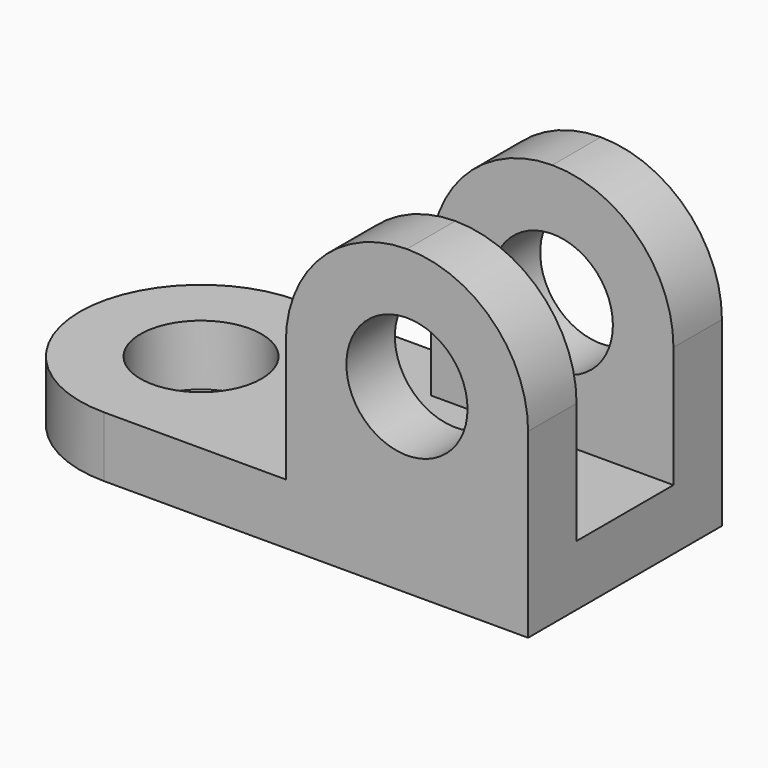
from build123d import *

# Parameters (mm, degrees)
F0_W      = 114.3
F0_H      = 63.5
F1_DEPTH  = 50.8
F2_W      = 25.4
F2_H      = 57.0441053795
F3_DEPTH  = 114.301
F4_W      = 63.5
F4_H      = 12.7
F5_DEPTH  = 50.8
F6_W      = 63.5
F6_H      = 12.7
F7_DEPTH  = 50.8
F8_R      = 12.7
F9_DEPTH  = 50.801
F10_R     = 25.39999
F11_R     = 12.7
F12_DEPTH = 12.701


# Not quite as in the source:
# - a fillet or chamfer is up to 0.001 mm smaller than in the source, because OpenCascade refuses the exact size


with BuildPart() as f1:
    # F0 (on Front) → F1 (new body)
    with BuildSketch(Plane.XZ):
        with Locations((5.5195242167, 20.4444855223)):
            Rectangle(F0_W, F0_H)
    extrude(amount=F1_DEPTH)

    # F2 (on face) → F3 (cut, through all)
    with BuildSketch(Plane.YZ.offset(62.6695242167)):
        with Locations((-25.4, 29.9165382121)):
            Rectangle(F2_W, F2_H)
    extrude(amount=-F3_DEPTH, mode=Mode.SUBTRACT)

    # F4 (on face) → F5 (cut)
    with BuildSketch(Plane.XY.offset(52.1944855223)):
        with Locations((-19.8804757833, -44.45)):
            Rectangle(F4_W, F4_H)
    extrude(amount=-F5_DEPTH, mode=Mode.SUBTRACT)

    # F6 (on face) → F7 (cut)
    with BuildSketch(Plane.XY.offset(52.1944855223)):
        with Locations((-19.8804757833, -6.35)):
            Rectangle(F6_W, F6_H)
    extrude(amount=-F7_DEPTH, mode=Mode.SUBTRACT)

    # F8 (on face) → F9 (cut, through all)
    with BuildSketch(Plane.XZ.offset(50.8)):
        with Locations((37.2695242167, 26.7944855223)):
            Circle(F8_R)
    extrude(amount=-F9_DEPTH, mode=Mode.SUBTRACT)

    # F10 (radius 25.4 in the source; OpenCascade refuses exactly that, so slightly less here)
    f10_edges = [f1.edges().sort_by_distance(p)[0] for p in [
        (62.669524, -44.45, 52.194486),
        (11.869524, -44.45, 52.194486),
        (11.869524, -6.35, 52.194486),
        (62.669524, -6.35, 52.194486),
        (-51.630476, -50.8, -4.955514),
        (-51.630476, 0, -4.955514),
    ]]
    fillet(f10_edges, radius=F10_R)

    # F11 (on face) → F12 (cut, through all)
    with BuildSketch(Plane.XY.offset(1.3944855223)):
        with Locations((-26.2304757833, -25.4)):
            Circle(F11_R)
    extrude(amount=-F12_DEPTH, mode=Mode.SUBTRACT)


solid = f1.part
